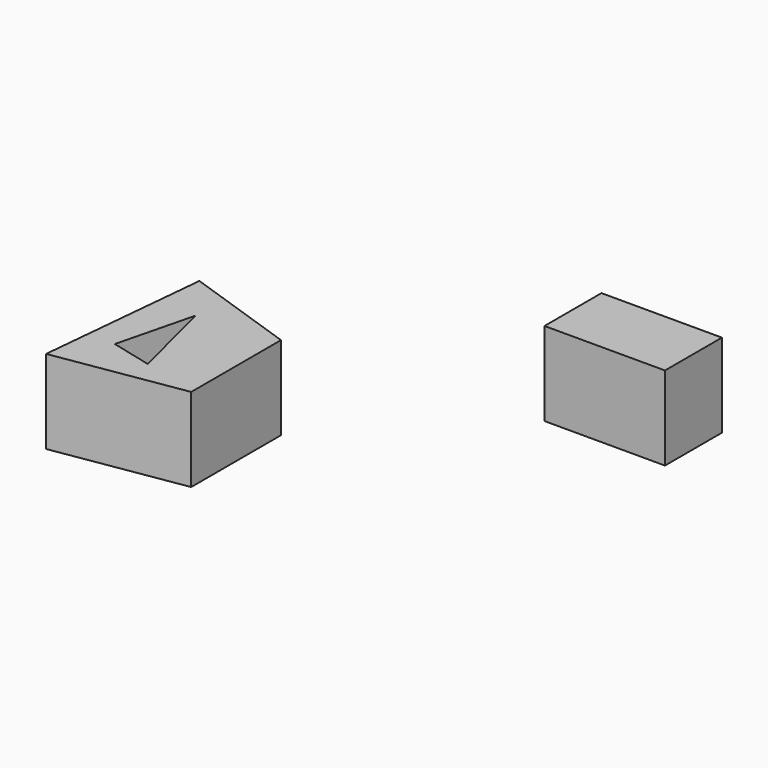
from build123d import *

# Parameters (mm, degrees)
F1_DEPTH = 25.4
F0_W     = 36.5379918367
F0_H     = 21.5906333178
F3_DEPTH = 25.4


# Not quite as in the source:
# - the program builds the solid bodies; features that only make, move or delete a surface that nothing else refers to are left out


with BuildPart() as f1:
    # F0 (on Top) → F1 (new body)
    with BuildSketch(Plane.XY):
        Polygon((-20.9524314851, -29.0797241032), (-54.9991987646, -17.4539964646), (-59.9816553295, -69.3545565009), (-20.9524314851, -63.1264895201), align=None)
        Polygon((-50.4319518805, -55.2375987172), (-44.6190871298, -31.9861508906), (-37.9269696142, -58.3638457864), align=None, mode=Mode.SUBTRACT)
    extrude(amount=F1_DEPTH)


with BuildPart() as f3:
    # F0 (on Top) → F3 (new body)
    with BuildSketch(Plane.XY):
        with Locations((41.5204456076, 26.3654785231)):
            Rectangle(F0_W, F0_H)
    extrude(amount=F3_DEPTH)


solid = Compound([f1.part, f3.part])
